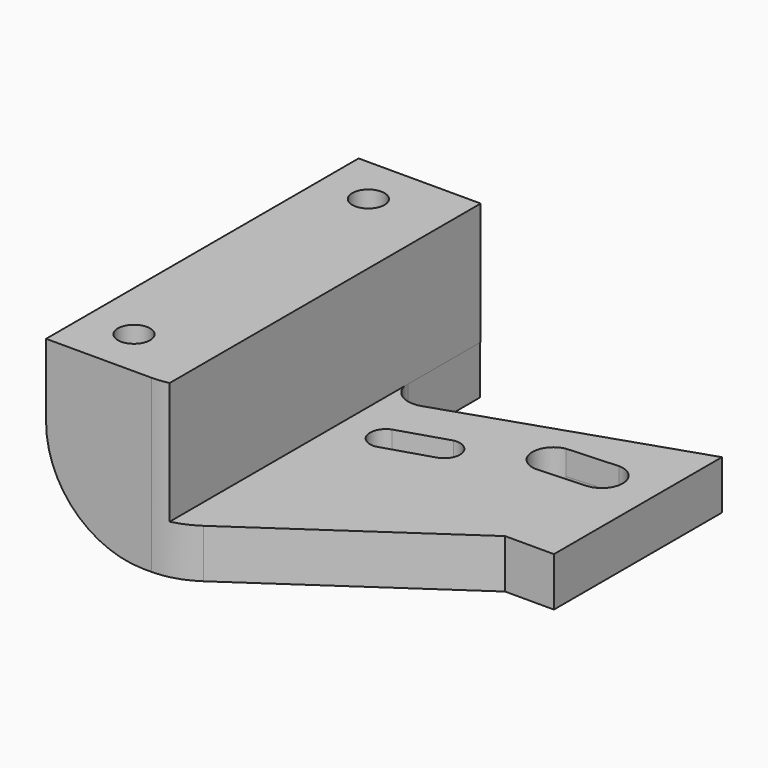
from build123d import *

# Parameters (mm, degrees)
F1_DEPTH     = 80
F2_R         = 3.3
F3_DEPTH     = 25
F5_DEPTH     = 25
F7_W         = 50
F7_H         = 5
F8_DEPTH     = 10
F9_DEPTH     = 25
F11_W        = 20
F11_H        = 80
F11_R        = 3.3
F12_DEPTH    = 30
F13_T1_DEPTH = 180
F15_DEPTH    = 5
F16_DEPTH    = 10
F17_R        = 15


# Not quite as in the source:
# - a fillet or chamfer that OpenCascade refuses, or shapes differently, is made with other operations: its cross-section is extruded or revolved along the edge and cut away or added


with BuildPart() as f1:
    # F0 (on Front) → F1 (new body)
    with BuildSketch(Plane.XZ):
        Polygon((25, 0), (0, 0), (0, -5), (20, -5), (20, -35), (70, -35), (70, -30), (25, -30), align=None)
    extrude(amount=F1_DEPTH)

    # F2 (on face) → F3 (cut)
    with BuildSketch(Plane(origin=(0, 0, -5), x_dir=(1, 0, 0), z_dir=(0, 0, -1))):
        with Locations((10, 70)):
            Circle(F2_R)
        with Locations((10, 10)):
            Circle(F2_R)
    extrude(amount=-F3_DEPTH, mode=Mode.SUBTRACT)

    # F4 (on face) → F5 (cut)
    with BuildSketch(Plane(origin=(0, 0, -35), x_dir=(1, 0, 0), z_dir=(0, 0, -1))):
        Polygon((26.251764968, 80), (70, 50), (70, 80), align=None)
    extrude(amount=-F5_DEPTH, mode=Mode.SUBTRACT)

    # F7 (on face) → F8 (join)
    with BuildSketch(Plane.YZ.offset(70)):
        with Locations((-25, -32.5)):
            Rectangle(F7_W, F7_H)
    extrude(amount=F8_DEPTH)

    # F6 (on face) → F9 (cut)
    with BuildSketch(Plane(origin=(0, 0, -35), x_dir=(1, 0, 0), z_dir=(0, 0, -1))):
        with BuildLine():
            Line((33.2249982655, 32.343756614), (42.1594857766, 29.5393376388))
            Line((42.1594857766, 29.5393376388), (42.9081277459, 29.3043486994))
            ThreePointArc((42.9081277459, 29.3043486994), (46.655005577, 31.7199744818), (44.4654424177, 35.6032919518))
            Line((44.4654424177, 35.6032919518), (35.4531247971, 38.407048043))
            Line((35.4531247971, 38.407048043), (34.4525012517, 38.7183447014))
            ThreePointArc((34.4525012517, 38.7183447014), (30.8539491948, 36.3153921333), (32.8322864897, 32.4670237129))
            Line((32.8322864897, 32.4670237129), (33.2249982655, 32.343756614))
        make_face()
        with BuildLine():
            Line((59.8621358425, 20.2152762479), (68.4127130059, 19.7402941432))
            Line((68.4127130059, 19.7402941432), (69.1118786564, 19.7014556922))
            ThreePointArc((69.1118786564, 19.7014556922), (69.558979499, 19.7364871386), (70, 19.8178952667))
            Line((70, 19.8178952667), (70, 28.1821047333))
            ThreePointArc((70, 28.1821047333), (69.6155307917, 28.2557163727), (69.2259603929, 28.2940589075))
            Line((69.2259603929, 28.2940589075), (59.7544017562, 28.7924677921))
            ThreePointArc((59.7544017562, 28.7924677921), (55.2347672319, 25.0457008651), (58.6655262733, 20.2817475657))
            Line((58.6655262733, 20.2817475657), (59.8621358425, 20.2152762479))
        make_face()
        with BuildLine():
            Line((70, 28.1821047333), (70, 19.8178952667))
            ThreePointArc((70, 19.8178952667), (73.3, 24), (70, 28.1821047333))
        make_face()
    extrude(amount=-F9_DEPTH, mode=Mode.SUBTRACT)

    # F11 (on face) → F12 (join)
    with BuildSketch(Plane(origin=(0, 0, -5), x_dir=(1, 0, 0), z_dir=(0, 0, -1))):
        with Locations((10, 40)):
            Rectangle(F11_W, F11_H)
        with Locations((10, 10)):
            Circle(F11_R, mode=Mode.SUBTRACT)
        with Locations((10, 70)):
            Circle(F11_R, mode=Mode.SUBTRACT)
    extrude(amount=F12_DEPTH)

    # F13: fillet of radius 20 on 1 edges, made by hand

    # F13_s2 → F13_t1 (cut)
    with BuildSketch(Plane.XZ.offset(-50)):
        with BuildLine():
            ThreePointArc((20, -35), (5.8578643763, -29.1421356237), (0, -15))
            Line((0, -15), (0, -35))
            Line((0, -35), (20, -35))
        make_face()
    extrude(amount=F13_T1_DEPTH, mode=Mode.SUBTRACT)

    # F14 (on face) → F15 (join)
    with BuildSketch(Plane.XY.offset(-30)):
        Polygon((80, 0), (25, 0), (25, -80), (26.251764968, -80), (70, -50), (80, -50), (80, -47.8473119438), align=None)
        with BuildLine():
            ThreePointArc((42.9081277459, -29.3043486994), (46.655005577, -31.7199744818), (44.4654424177, -35.6032919518))
            Line((44.4654424177, -35.6032919518), (34.4525012517, -38.7183447014))
            ThreePointArc((34.4525012517, -38.7183447014), (30.8539491948, -36.3153921333), (32.8322864897, -32.4670237129))
            Line((32.8322864897, -32.4670237129), (42.9081277459, -29.3043486994))
        make_face(mode=Mode.SUBTRACT)
        with BuildLine():
            ThreePointArc((69.1118786564, -19.7014556922), (73.2996210658, -23.9429150602), (69.2259603929, -28.2940589075))
            Line((69.2259603929, -28.2940589075), (59.7544017562, -28.7924677921))
            ThreePointArc((59.7544017562, -28.7924677921), (55.2347672319, -25.0457008651), (58.6655262733, -20.2817475657))
            Line((58.6655262733, -20.2817475657), (69.1118786564, -19.7014556922))
        make_face(mode=Mode.SUBTRACT)
    extrude(amount=F15_DEPTH)

    # F10 (on face) → F16 (cut)
    with BuildSketch(Plane(origin=(0, 0, -35), x_dir=(1, 0, 0), z_dir=(0, 0, -1))):
        with BuildLine():
            Line((80, 7), (31.4644035058, 23.1785321647))
            ThreePointArc((31.4644035058, 23.1785321647), (26.9597132524, 22.4913266004), (24.8832646757, 18.4351156745))
            Line((24.8832646757, 18.4351156745), (24.8832646757, 0))
            Line((24.8832646757, 0), (80, 0))
            Line((80, 0), (80, 7))
        make_face()
    extrude(amount=-F16_DEPTH, mode=Mode.SUBTRACT)

    # F17
    f17_edges = [f1.edges().sort_by_distance(p)[0] for p in [
        (26.251765, -80, -30),
    ]]
    fillet(f17_edges, radius=F17_R)


solid = f1.part
